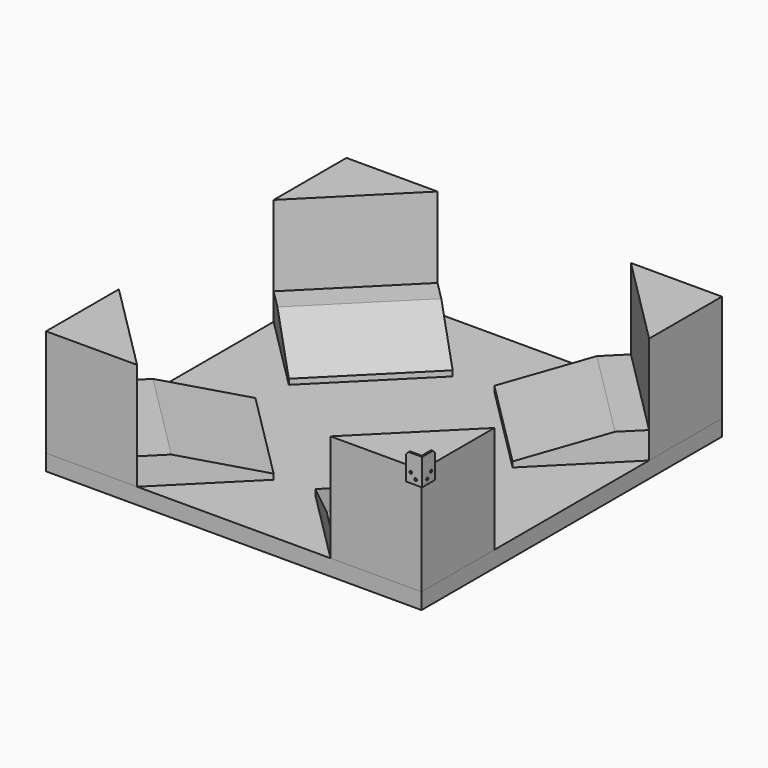
from build123d import *

# Parameters (mm, degrees)
F0_W           = 700
F0_H           = 700
F1_DEPTH       = 30
F3_DEPTH       = 200
F6_DEPTH       = 240
F8_ANGLE       = 90
F9_ANGLE       = 180
F10_ANGLE      = 270
F11_ANGLE      = 90
F12_ANGLE      = 180
F13_ANGLE      = 270
F15_DEPTH      = 25
F15_DEPTH_BACK = 25
F17_R          = 2.5
F18_DEPTH      = 25
F16_R          = 2.5
F19_DEPTH      = 25
F20_SIZE       = 5


with BuildPart() as f1:
    # F0 (on Top) → F1 (new body)
    with BuildSketch(Plane.XY):
        Rectangle(F0_W, F0_H)
    extrude(amount=-F1_DEPTH)


with BuildPart() as f3:
    # F2 (on face) → F3 (new body)
    with BuildSketch(Plane.XY):
        Polygon((-180.3300858899, -350), (-350, -180.3300858899), (-350, -350), align=None)
    extrude(amount=F3_DEPTH)


with BuildPart() as f6:
    # F5 (on face) → F6 (new body)
    with BuildSketch(Plane(origin=(84.834957055, -84.834957055, 0), x_dir=(-0.7071067812, -0.7071067812, 0), z_dir=(-0.7071067812, 0.7071067812, 0))):
        Polygon((375, 0), (375, 50), (325, 50), (175, 10), (175, 0), align=None)
    extrude(amount=F6_DEPTH)


with BuildPart() as f8_1:
    # F8: copy of F3
    add(f3.part.rotate(Axis((0, 0, 150), (0, 0, 1)), F8_ANGLE))


with BuildPart() as f9_1:
    # F9: copy of F3
    add(f3.part.rotate(Axis((0, 0, 150), (0, 0, 1)), F9_ANGLE))


with BuildPart() as f10_1:
    # F10: copy of F3
    add(f3.part.rotate(Axis((0, 0, 150), (0, 0, 1)), F10_ANGLE))


with BuildPart() as f11_1:
    # F11: copy of F6
    add(f6.part.rotate(Axis((0, 0, 150), (0, 0, 1)), F11_ANGLE))


with BuildPart() as f12_1:
    # F12: copy of F6
    add(f6.part.rotate(Axis((0, 0, 150), (0, 0, 1)), F12_ANGLE))


with BuildPart() as f13_1:
    # F13: copy of F6
    add(f6.part.rotate(Axis((0, 0, 150), (0, 0, 1)), F13_ANGLE))


with BuildPart() as f15:
    # F14 (on face) → F15 (new body, two sides)
    with BuildSketch(Plane.XY.offset(200)) as f15_sk:
        Polygon((355, -325), (352, -325), (352, -352), (325, -352), (325, -355), (355, -355), align=None)
    extrude(amount=F15_DEPTH)
    extrude(f15_sk.sketch, amount=-F15_DEPTH_BACK)

    # F17 (on face) → F18 (cut)
    with BuildSketch(Plane.YZ.offset(355)):
        with Locations((-334, 193)):
            Circle(F17_R)
        with Locations((-343, 184)):
            Circle(F17_R)
    extrude(amount=-F18_DEPTH, mode=Mode.SUBTRACT)

    # F16 (on face) → F19 (cut)
    with BuildSketch(Plane.XZ.offset(355)):
        with Locations((334, 193)):
            Circle(F16_R)
        with Locations((343, 184)):
            Circle(F16_R)
    extrude(amount=-F19_DEPTH, mode=Mode.SUBTRACT)

    # F20
    f20_edges = [f15.edges().sort_by_distance(p)[0] for p in [
        (325, -353.5, 225),
        (353.5, -325, 225),
    ]]
    chamfer(f20_edges, length=F20_SIZE)


solid = Compound([f1.part, f3.part, f6.part, f8_1.part, f9_1.part, f10_1.part, f11_1.part, f12_1.part, f13_1.part, f15.part])
